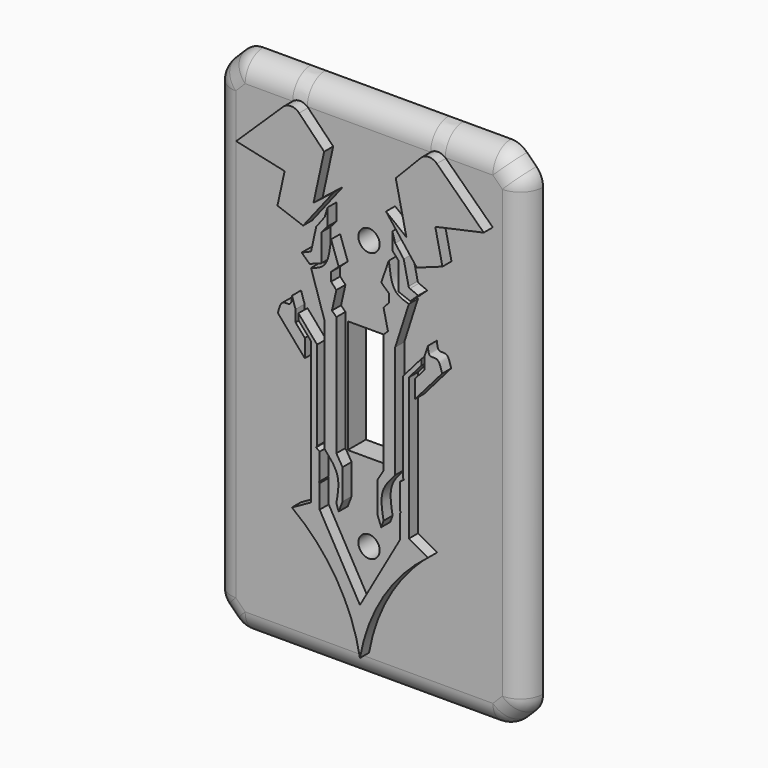
from build123d import *

# Parameters (mm, degrees)
F0_W     = 69.85
F0_H     = 114.3
F0_R     = 2.3876
F0_W_2   = 9.525
F0_H_2   = 25.4
F1_DEPTH = 5.08
F2_SIZE  = 5.08
F4_DEPTH = 2.54
F5_R     = 5.08
F6_R     = 5.07999


# Not quite as in the source:
# - a fillet or chamfer is up to 0.001 mm smaller than in the source, because OpenCascade refuses the exact size


with BuildPart() as f1:
    # F0 (on Front) → F1 (new body)
    with BuildSketch(Plane.XZ):
        Rectangle(F0_W, F0_H)
        with Locations((0, -30.1625)):
            Circle(F0_R, mode=Mode.SUBTRACT)
        Rectangle(F0_W_2, F0_H_2, mode=Mode.SUBTRACT)
        with Locations((0, 30.1625)):
            Circle(F0_R, mode=Mode.SUBTRACT)
    extrude(amount=F1_DEPTH)

    # F2
    f2_edges = [f1.edges().sort_by_distance(p)[0] for p in [
        (-34.925, -2.54, -57.15),
        (34.925, -2.54, -57.15),
        (34.925, -2.54, 57.15),
        (-34.925, -2.54, 57.15),
    ]]
    chamfer(f2_edges, length=F2_SIZE)

    # F3 (on face) → F4 (join)
    with BuildSketch(Plane.XZ.offset(5.08)):
        with BuildLine():
            Line((-10.9491456177, -24.015756105), (-15.24, -26.3939449695))
            ThreePointArc((-15.24, -26.3939449695), (-5.2454326853, -37.2936038704), (0, -51.1203669012))
            ThreePointArc((0, -51.1203669012), (5.2454326853, -37.2936038704), (15.24, -26.3939449695))
            Line((15.24, -26.3939449695), (10.9491456177, -24.015756105))
            Line((10.9491456177, -24.015756105), (10.9491456177, 7.7689122409))
            Line((10.9491456177, 7.7689122409), (13.7791661546, 11.0349841416))
            Line((13.7791661546, 11.0349841416), (13.7791661546, 12.3685728759))
            Line((13.7791661546, 12.3685728759), (9.6029456177, 7.5488776231))
            Line((9.6029456177, 7.5488776231), (9.6029456177, -12.4826692045))
            Line((9.6029456177, -12.4826692045), (9.8263714463, -12.7935418859))
            Line((9.8263714463, -12.7935418859), (9.0244112121, -13.3699149172))
            Line((9.0244112121, -13.3699149172), (9.0244112121, -19.2372985184))
            Line((9.0244112121, -19.2372985184), (9.1956509277, -19.3663351238))
            Line((9.1956509277, -19.3663351238), (9.0244112121, -19.593581029))
            Line((9.0244112121, -19.593581029), (9.0244112121, -24.8032323161))
            Line((9.0244112121, -24.8032323161), (0, -40.6771302223))
            Line((0, -40.6771302223), (-9.0244112121, -24.8032323161))
            Line((-9.0244112121, -24.8032323161), (-9.0244112121, -19.593581029))
            Line((-9.0244112121, -19.593581029), (-9.1956509277, -19.3663351238))
            Line((-9.1956509277, -19.3663351238), (-9.0244112121, -19.2372985184))
            Line((-9.0244112121, -19.2372985184), (-9.0244112121, -13.3699149172))
            Line((-9.0244112121, -13.3699149172), (-9.8263714463, -12.7935418859))
            Line((-9.8263714463, -12.7935418859), (-9.6029456177, -12.4826692045))
            Line((-9.6029456177, -12.4826692045), (-9.6029456177, 7.5488776231))
            Line((-9.6029456177, 7.5488776231), (-13.7791661546, 12.3685728759))
            Line((-13.7791661546, 12.3685728759), (-13.7791661546, 11.0349841416))
            Line((-13.7791661546, 11.0349841416), (-10.9491456177, 7.7689122409))
            Line((-10.9491456177, 7.7689122409), (-10.9491456177, -24.015756105))
        make_face()
        with BuildLine():
            Line((15.2168534696, 15.3767615557), (14.430125244, 12.9491025582))
            Line((14.430125244, 12.9491025582), (14.430125244, 10.3672910482))
            Line((14.430125244, 10.3672910482), (12.3528247342, 7.969918755))
            Line((12.3528247342, 7.969918755), (12.3528247342, 3.9576585405))
            Line((12.3528247342, 3.9576585405), (18.4005603076, 10.9372330566))
            add(Edge.make_bspline(
                [(18.4005603076, 10.9372330566), (18.1233475721, 12.0101345827), (17.6392451583, 13.8837650195), (15.3663734292, 13.1144073025), (15.2684691915, 14.5957752031), (15.2168534696, 15.3767615557)],
                knots=[0, 0, 0, 0, 0.3878172967, 0.6772534788, 1, 1, 1, 1], degree=3))
        make_face()
        with BuildLine():
            Line((-12.3528247342, 3.9576585405), (-12.3528247342, 7.969918755))
            Line((-12.3528247342, 7.969918755), (-14.430125244, 10.3672910482))
            Line((-14.430125244, 10.3672910482), (-14.430125244, 12.9491025582))
            Line((-14.430125244, 12.9491025582), (-15.2168534696, 15.3767615557))
            add(Edge.make_bspline(
                [(-18.4005603076, 10.9372330566), (-18.1233475721, 12.0101345827), (-17.6392451583, 13.8837650195), (-15.3663734292, 13.1144073025), (-15.2684691915, 14.5957752031), (-15.2168534696, 15.3767615557)],
                knots=[0, 0, 0, 0, 0.3878172967, 0.6772534788, 1, 1, 1, 1], degree=3))
            Line((-18.4005603076, 10.9372330566), (-12.3528247342, 3.9576585405))
        make_face()
        with BuildLine():
            Line((-7.9025151208, 12.7211911604), (-7.9025151208, -12.4826692045))
            add(Edge.make_bspline(
                [(-7.9025151208, -12.4826692045), (-6.7088471029, -13.8130212346), (-4.2657929258, -16.5358235846), (-4.9393104998, -20.3774464422), (-5.2837496623, -22.3420653492)],
                knots=[0, 0, 0, 0, 0.4885966218, 1, 1, 1, 1], degree=3))
            Line((-5.2837496623, -22.3420653492), (-4.7625, -23.7969346344))
            Line((-4.7625, -23.7969346344), (-3.9016241208, -21.5418860316))
            Line((-3.9016241208, -21.5418860316), (-3.9016241208, -14.7672407329))
            Line((-3.9016241208, -14.7672407329), (-5.2837496623, -12.4826692045))
            Line((-5.2837496623, -12.4826692045), (-5.2837496623, 14.3719073385))
            Line((-5.2837496623, 14.3719073385), (-6.2687969767, 15.3429154307))
            Line((-6.2687969767, 15.3429154307), (-5.2837496623, 19.7124555707))
            Line((-5.2837496623, 19.7124555707), (-6.4629982226, 20.974766463))
            Line((-6.4629982226, 20.974766463), (-6.4629982226, 22.91678451))
            Line((-6.4629982226, 22.91678451), (-4.7625, 24.4703982025))
            Line((-4.7625, 24.4703982025), (-6.4629982226, 29.3254423887))
            add(Edge.make_bspline(
                [(-6.4629982226, 29.3254423887), (-6.7147913988, 27.2015270399), (-7.1642091406, 23.4106171591), (-9.7931216323, 22.5955100704), (-10.9491456177, 22.237079218)],
                knots=[0, 0, 0, 0, 0.560265323, 1, 1, 1, 1], degree=3))
            Line((-10.9491456177, 22.237079218), (-7.9025151208, 12.7211911604))
        make_face()
        with BuildLine():
            Line((6.4629982226, 20.974766463), (5.2837496623, 19.7124555707))
            Line((5.2837496623, 19.7124555707), (6.2687969767, 15.3429154307))
            Line((6.2687969767, 15.3429154307), (5.2837496623, 14.3719073385))
            Line((5.2837496623, 14.3719073385), (5.2837496623, -12.4826692045))
            Line((5.2837496623, -12.4826692045), (3.9016241208, -14.7672407329))
            Line((3.9016241208, -14.7672407329), (3.9016241208, -21.5418860316))
            Line((3.9016241208, -21.5418860316), (4.7625, -23.7969346344))
            Line((4.7625, -23.7969346344), (5.2837496623, -22.3420653492))
            add(Edge.make_bspline(
                [(7.9025151208, -12.4826692045), (6.7088471029, -13.8130212346), (4.2657929258, -16.5358235846), (4.9393104998, -20.3774464422), (5.2837496623, -22.3420653492)],
                knots=[0, 0, 0, 0, 0.4885966218, 1, 1, 1, 1], degree=3))
            Line((7.9025151208, -12.4826692045), (7.9025151208, 12.7211911604))
            Line((7.9025151208, 12.7211911604), (10.9491456177, 22.237079218))
            add(Edge.make_bspline(
                [(6.4629982226, 29.3254423887), (6.7147913988, 27.2015270399), (7.1642091406, 23.4106171591), (9.7931216323, 22.5955100704), (10.9491456177, 22.237079218)],
                knots=[0, 0, 0, 0, 0.560265323, 1, 1, 1, 1], degree=3))
            Line((6.4629982226, 29.3254423887), (4.7625, 24.4703982025))
            Line((4.7625, 24.4703982025), (6.4629982226, 22.91678451))
            Line((6.4629982226, 22.91678451), (6.4629982226, 20.974766463))
        make_face()
        with BuildLine():
            Line((8.664281252, 23.8877926022), (11.2787401304, 22.91678451))
            Line((11.2787401304, 22.91678451), (13.051327318, 24.5748348534))
            Line((13.051327318, 24.5748348534), (11.1917219018, 25.3588579305))
            ThreePointArc((11.1917219018, 25.3588579305), (10.9984776228, 25.5021521413), (10.8928335564, 25.7182907854))
            Line((10.8928335564, 25.7182907854), (9.7931216323, 30.7403579354))
            Line((9.7931216323, 30.7403579354), (7.9025151208, 33.2289571039))
            Line((7.9025151208, 33.2289571039), (7.249711547, 35.3622324765))
            Line((7.249711547, 35.3622324765), (7.249711547, 31.6020064056))
            Line((7.249711547, 31.6020064056), (8.664281252, 30.0072413649))
            Line((8.664281252, 30.0072413649), (8.664281252, 23.8877926022))
        make_face()
        with BuildLine():
            Line((-13.051327318, 24.5748348534), (-11.2787401304, 22.91678451))
            Line((-11.2787401304, 22.91678451), (-8.664281252, 23.8877926022))
            Line((-8.664281252, 23.8877926022), (-8.664281252, 30.0072413649))
            Line((-8.664281252, 30.0072413649), (-7.249711547, 31.6020064056))
            Line((-7.249711547, 31.6020064056), (-7.249711547, 35.3622324765))
            Line((-7.249711547, 35.3622324765), (-7.9025151208, 33.2289571039))
            Line((-7.9025151208, 33.2289571039), (-9.7931216323, 30.7403579354))
            Line((-9.7931216323, 30.7403579354), (-10.8928335564, 25.7182907854))
            ThreePointArc((-10.8928335564, 25.7182907854), (-10.9984776228, 25.5021521413), (-11.1917219018, 25.3588579305))
            Line((-11.1917219018, 25.3588579305), (-13.051327318, 24.5748348534))
        make_face()
        with BuildLine():
            Line((-18.4751220397, 32.062277317), (-12.7323835574, 29.9877415643))
            Line((-12.7323835574, 29.9877415643), (-5.8382207013, 38.8251322554))
            Line((-5.8382207013, 38.8251322554), (-10.4019630186, 35.2319072233))
            Line((-10.4019630186, 35.2319072233), (-8.0194973537, 46.1119407026))
            Line((-8.0194973537, 46.1119407026), (-13.6249894716, 51.8940991802))
            ThreePointArc((-13.6249894716, 51.8940991802), (-15.4092844735, 52.6658187712), (-17.216659725, 51.9498198316))
            Line((-17.216659725, 51.9498198316), (-27.7217694612, 41.7656801108))
            Line((-27.7217694612, 41.7656801108), (-24.3511985749, 41.0276061496))
            Line((-24.3511985749, 41.0276061496), (-16.870627516, 39.389540997))
            Line((-16.870627516, 39.389540997), (-18.4751220397, 32.062277317))
        make_face()
        with BuildLine():
            Line((8.0194973537, 46.1119407026), (10.4019630186, 35.2319072233))
            Line((10.4019630186, 35.2319072233), (5.8382207013, 38.8251322554))
            Line((5.8382207013, 38.8251322554), (12.7323835574, 29.9877415643))
            Line((12.7323835574, 29.9877415643), (18.4751220397, 32.062277317))
            Line((18.4751220397, 32.062277317), (16.870627516, 39.389540997))
            Line((16.870627516, 39.389540997), (24.3511985749, 41.0276061496))
            Line((24.3511985749, 41.0276061496), (27.7217694612, 41.7656801108))
            Line((27.7217694612, 41.7656801108), (17.216659725, 51.9498198316))
            ThreePointArc((17.216659725, 51.9498198316), (15.4092844735, 52.6658187712), (13.6249894716, 51.8940991802))
            Line((13.6249894716, 51.8940991802), (8.0194973537, 46.1119407026))
        make_face()
    extrude(amount=F4_DEPTH)

    # F5
    f5_edges = [f1.edges().sort_by_distance(p)[0] for p in [
        (29.845, -2.54, 57.15),
        (34.925, -2.54, 52.07),
        (-29.845, -2.54, 57.15),
        (-34.925, -2.54, 52.07),
        (-34.925, -2.54, -52.07),
        (-29.845, -2.54, -57.15),
        (29.845, -2.54, -57.15),
        (34.925, -2.54, -52.07),
    ]]
    fillet(f5_edges, radius=F5_R)

    # F6 (radius 5.08 in the source; OpenCascade refuses exactly that, so slightly less here)
    f6_edges = [f1.edges().sort_by_distance(p)[0] for p in [
        (34.925, -5.08, 0),
    ]]
    fillet(f6_edges, radius=F6_R)


solid = f1.part
